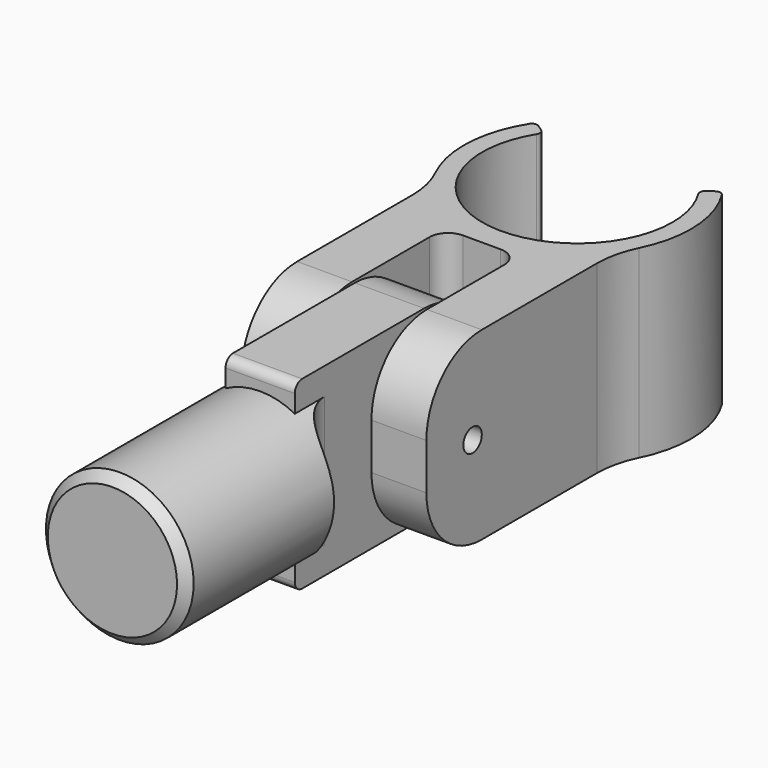
from build123d import *

# Parameters (mm, degrees)
F1_DEPTH      = 12.7
F0_W          = 7.5565
F0_H          = 25.4
F2_DEPTH      = 12.7
F3_T1_DEPTH   = 25.4
F3_T3_DEPTH   = 12.7
F3_T5_DEPTH   = 12.7
F4_R          = 0.762
F5_W          = 31.75
F5_H          = 25.4
F5_R          = 1.5875
F6_DEPTH      = 4.7625
F7_DEPTH      = 25.4
F7_DEPTH_BACK = 25.4
F8_R          = 10.16
F9_DEPTH      = 25.4
F10_R         = 9.525
F10_2_R       = 9.525
F11_T4_DEPTH  = 43.3492834119
F11_S5_R      = 10.16
F11_T6_DEPTH  = 23
F11_T10_DEPTH = 43.3492834119
F11_S11_R     = 10.16
F11_T12_DEPTH = 23
F12_R         = 1.27
F13_R         = 2.54
F14_SIZE      = 1.27


# Not quite as in the source:
# - a fillet or chamfer that OpenCascade refuses, or shapes differently, is made with other operations: its cross-section is extruded or revolved along the edge and cut away or added


with BuildPart() as f1:
    # F0 (on Top) → F1 (new body, symmetric)
    with BuildSketch(Plane.XY):
        with BuildLine():
            ThreePointArc((12.7, -9.0953637091), (14.8728333044, -4.7764495705), (15.621, 0))
            ThreePointArc((15.621, 0), (14.8980124876, 4.6973252941), (12.7959740838, 8.9598375122))
            Line((12.7959740838, 8.9598375122), (10.7153278913, 7.5029533639))
            ThreePointArc((10.7153278913, 7.5029533639), (12.4755714327, 3.9335325633), (13.081, 0))
            ThreePointArc((13.081, 0), (-3.9335325633, -12.4755714327), (-10.7153278913, 7.5029533639))
            Line((-10.7153278913, 7.5029533639), (-12.7959740838, 8.9598375122))
            ThreePointArc((-12.7959740838, 8.9598375122), (-15.6207793149, -0.0830336901), (-12.7, -9.0953637091))
            ThreePointArc((-12.7, -9.0953637091), (0, -15.621), (12.7, -9.0953637091))
        make_face()
    extrude(amount=F1_DEPTH, both=True)

    # F0 (on Top) → F2 (join, symmetric)
    with BuildSketch(Plane.XY):
        with BuildLine():
            Line((12.7, -16.4338), (12.7, -9.0953637091))
            ThreePointArc((12.7, -9.0953637091), (0, -15.621), (-12.7, -9.0953637091))
            Line((-12.7, -9.0953637091), (-12.7, -16.4338))
            Line((-12.7, -16.4338), (-5.1435, -16.4338))
            Line((-5.1435, -16.4338), (5.1435, -16.4338))
            Line((5.1435, -16.4338), (12.7, -16.4338))
        make_face()
        with Locations((-8.92175, -29.1338)):
            Rectangle(F0_W, F0_H)
        with Locations((8.92175, -29.1338)):
            Rectangle(F0_W, F0_H)
    extrude(amount=F2_DEPTH, both=True)

    # F3: fillet of radius 12.7 on 3 edges, made by hand

    # F3_s2 → F3_t1 (join)
    with BuildSketch(Plane.XY.offset(-12.7)):
        with BuildLine():
            ThreePointArc((-14.0098654709, -6.9093639714), (-13.0318006864, -9.6427001587), (-12.7, -12.5267330538))
            Line((-12.7, -12.5267330538), (-12.7, -9.0953637091))
            ThreePointArc((-12.7, -9.0953637091), (-13.3995849593, -8.0291197475), (-14.0098654709, -6.9093639714))
        make_face()
    extrude(amount=F3_T1_DEPTH)

    # F3_s4 → F3_t3 (join)
    with BuildSketch(Plane.XY):
        with BuildLine():
            ThreePointArc((14.0098654709, -6.9093639714), (13.0318006864, -9.6427001587), (12.7, -12.5267330538))
            Line((12.7, -12.5267330538), (12.7, -9.0953637091))
            ThreePointArc((12.7, -9.0953637091), (13.3995849593, -8.0291197475), (14.0098654709, -6.9093639714))
        make_face()
    extrude(amount=F3_T3_DEPTH)

    # F3_s6 → F3_t5 (join)
    with BuildSketch(Plane.XY.offset(-12.7)):
        with BuildLine():
            ThreePointArc((12.7, -12.5267330538), (13.0318006864, -9.6427001587), (14.0098654709, -6.9093639714))
            ThreePointArc((14.0098654709, -6.9093639714), (13.3995849593, -8.0291197475), (12.7, -9.0953637091))
            Line((12.7, -9.0953637091), (12.7, -12.5267330538))
        make_face()
    extrude(amount=F3_T5_DEPTH)

    # F4
    f4_edges = [f1.edges().sort_by_distance(p)[0] for p in [
        (-12.795974, 8.959838, 0),
        (-10.715328, 7.502953, -6.35),
        (-10.715328, 7.502953, 6.35),
        (12.795974, 8.959838, 6.35),
        (12.795974, 8.959838, -6.35),
        (10.715328, 7.502953, 6.35),
        (10.715328, 7.502953, -6.35),
    ]]
    fillet(f4_edges, radius=F4_R)

    # F5 (on Right) → F7 (cut, two sides)
    with BuildSketch(Plane.YZ) as f7_sk:
        with Locations((-33.8963, 0)):
            Circle(F5_R)
    extrude(amount=-F7_DEPTH, mode=Mode.SUBTRACT)
    extrude(f7_sk.sketch, amount=F7_DEPTH_BACK, mode=Mode.SUBTRACT)

    # F10
    f10_edges = [f1.edges().sort_by_distance(p)[0] for p in [
        (8.92175, -41.8338, -12.7),
        (-8.92175, -41.8338, -12.7),
        (8.92175, -41.8338, 12.7),
        (-8.92175, -41.8338, 12.7),
    ]]
    fillet(f10_edges, radius=F10_R)

    # F13
    f13_edges = [f1.edges().sort_by_distance(p)[0] for p in [
        (5.1435, -16.4338, 0),
        (-5.1435, -16.4338, 0),
    ]]
    fillet(f13_edges, radius=F13_R)


with BuildPart() as f6:
    # F5 (on Right) → F6 (new body, symmetric)
    with BuildSketch(Plane.YZ):
        with Locations((-38.6588, 0)):
            Rectangle(F5_W, F5_H)
        with Locations((-33.8963, 0)):
            Circle(F5_R, mode=Mode.SUBTRACT)
    extrude(amount=F6_DEPTH, both=True)

    # F8 (on face) → F9 (join)
    with BuildSketch(Plane.XZ.offset(54.5338)):
        Circle(F8_R)
    extrude(amount=F9_DEPTH)

    # F10#2
    f10_2_edges = [f6.edges().sort_by_distance(p)[0] for p in [
        (0, -22.7838, -12.7),
        (0, -22.7838, 12.7),
    ]]
    fillet(f10_2_edges, radius=F10_2_R)

    # F11: fillet of radius 5.08 on 6 edges, made by hand


with BuildPart() as f11_tool2:
    # F11_s3 → F11_t4 (new body)
    with BuildSketch(Plane.XY.offset(21.6746417059)):
        with BuildLine():
            ThreePointArc((-4.7625, -49.4538), (-6.2503975516, -53.0459024484), (-9.8425, -54.5338))
            Line((-9.8425, -54.5338), (-4.7625, -54.5338))
            Line((-4.7625, -54.5338), (-4.7625, -49.4538))
        make_face()
    extrude(amount=-F11_T4_DEPTH)

    # F11_s5 → F11_t6 (intersect, symmetric)
    with BuildSketch(Plane.XZ.offset(52)):
        Circle(F11_S5_R)
    extrude(amount=F11_T6_DEPTH, both=True, mode=Mode.INTERSECT)


with BuildPart() as f6_1:
    add(f6.part)

    # F11_t1: union F11_tool2
    add(f11_tool2.part)


with BuildPart() as f11_tool8:
    # F11_s9 → F11_t10 (new body)
    with BuildSketch(Plane.XY.offset(21.6746417059)):
        with BuildLine():
            ThreePointArc((4.7625, -49.4538), (6.2503975516, -53.0459024484), (9.8425, -54.5338))
            Line((9.8425, -54.5338), (4.7625, -54.5338))
            Line((4.7625, -54.5338), (4.7625, -49.4538))
        make_face()
    extrude(amount=-F11_T10_DEPTH)

    # F11_s11 → F11_t12 (intersect, symmetric)
    with BuildSketch(Plane.XZ.offset(52)):
        Circle(F11_S11_R)
    extrude(amount=F11_T12_DEPTH, both=True, mode=Mode.INTERSECT)


with BuildPart() as f6_2:
    add(f6_1.part)

    # F11_t7: union F11_tool8
    add(f11_tool8.part)

    # F12
    f12_edges = [f6_2.edges().sort_by_distance(p)[0] for p in [
        (0, -54.5338, 12.7),
        (0, -54.5338, -12.7),
    ]]
    fillet(f12_edges, radius=F12_R)

    # F14
    f14_edges = [f6_2.edges().sort_by_distance(p)[0] for p in [
        (-10.16, -79.9338, 0),
    ]]
    chamfer(f14_edges, length=F14_SIZE)


solid = Compound([f1.part, f6_2.part])
